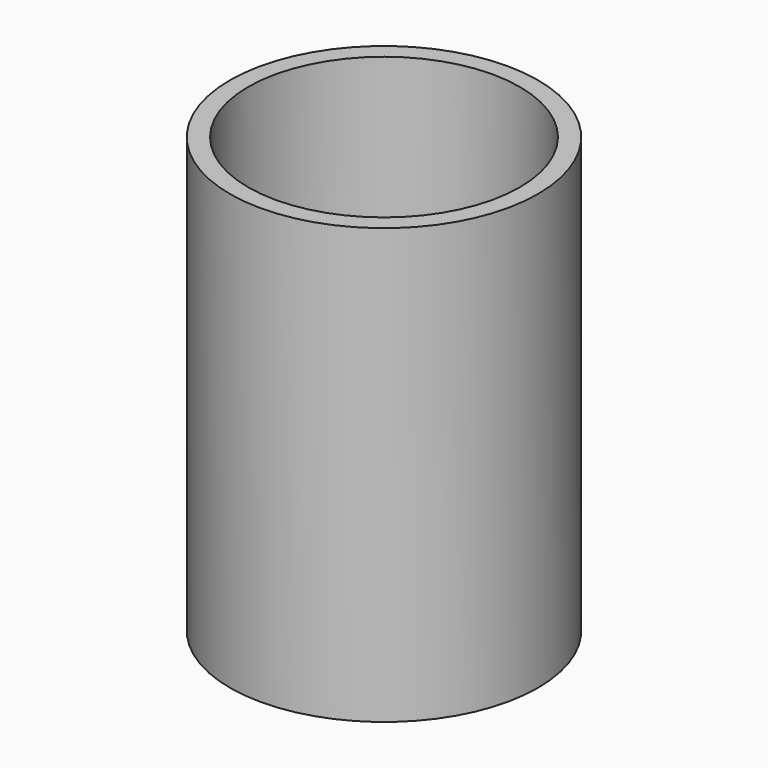
from build123d import *

# Parameters (mm, degrees)
F0_R     = 36.0004076963
F0_R_2   = 31.75
F1_DEPTH = 101.6
F2_R     = 36.0004076963
F2_R_2   = 32.3100361714
F2_R_3   = 31.75
F3_DEPTH = 13.716


with BuildPart() as f1:
    # F0 (on Top) → F1 (new body)
    with BuildSketch(Plane.XY):
        Circle(F0_R)
        Circle(F0_R_2, mode=Mode.SUBTRACT)
    extrude(amount=F1_DEPTH)

    # F2 (on face) → F3 (join)
    with BuildSketch(Plane(origin=(0, 0, 0), x_dir=(1, 0, 0), z_dir=(0, 0, -1))):
        Circle(F2_R)
        Circle(F2_R_2, mode=Mode.SUBTRACT)
        Circle(F2_R_2)
        Circle(F2_R_3, mode=Mode.SUBTRACT)
        Circle(F2_R_3)
    extrude(amount=-F3_DEPTH)


solid = f1.part
